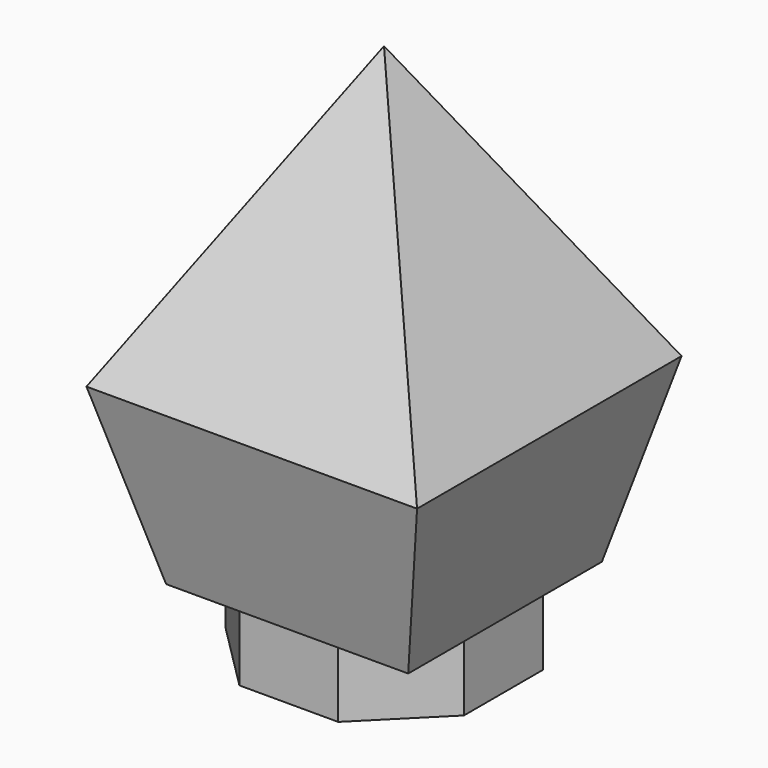
from build123d import *

# Parameters (mm, degrees)
F0_W        = 25
F0_H        = 25
F0_R        = 7.5
F1_DEPTH    = 35
F2_DEPTH    = 15
F3_SIZE2    = 21.650625
F3_SIZE     = 12.49999
F4_R        = 7.5
F5_DEPTH    = 5
F6_T1_DEPTH = 95.1228407313
F6_T3_DEPTH = 95.1228407313


# Not quite as in the source:
# - a fillet or chamfer that OpenCascade refuses, or shapes differently, is made with other operations: its cross-section is extruded or revolved along the edge and cut away or added
# - a fillet or chamfer is up to 0.001 mm smaller than in the source, because OpenCascade refuses the exact size


with BuildPart() as f1:
    # F0 (on Top) → F1 (new body)
    with BuildSketch(Plane.XY):
        with Locations((-12.5, -12.5)):
            Rectangle(F0_W, F0_H)
        with Locations((-12.5, -12.5)):
            Circle(F0_R, mode=Mode.SUBTRACT)
        with Locations((-12.5, -12.5)):
            Circle(F0_R)
    extrude(amount=F1_DEPTH)

    # F0 (on Top) → F2 (cut)
    with BuildSketch(Plane.XY):
        with Locations((-12.5, -12.5)):
            Circle(F0_R)
    extrude(amount=F2_DEPTH, mode=Mode.SUBTRACT)

    # F3 (size 12.5 and 21.6506350946 in the source; OpenCascade refuses exactly that, so slightly less here)
    f3_edges = [f1.edges().sort_by_distance(p)[0] for p in [
        (-25, -12.5, 35),
        (-12.5, -25, 35),
        (0, -12.5, 35),
        (-12.5, 0, 35),
    ]]
    f3_side = f1.faces().sort_by_distance((-12.5, -12.5, 35))[0]
    chamfer(f3_edges, length=F3_SIZE, length2=F3_SIZE2, reference=f3_side)

    # F4 (on Top) → F5 (join)
    with BuildSketch(Plane.XY):
        Polygon((-3.4594764784, -16.2579490188), (-3.4594764784, -8.802104896), (-8.731554417, -3.5300269574), (-16.1873985398, -3.5300269574), (-21.4594764784, -8.802104896), (-21.4594764784, -16.2579490188), (-16.1873985398, -21.5300269574), (-8.731554417, -21.5300269574), align=None)
        with Locations((-12.4594764784, -12.5300269574)):
            Circle(F4_R, mode=Mode.SUBTRACT)
    extrude(amount=-F5_DEPTH)

    # F6: chamfer of 13.5 x 3.3659280384 on 4 edges, made by hand

    # F6_s2 → F6_t1 (cut)
    with BuildSketch(Plane.YZ.offset(-60.0614203657)):
        Polygon((-25, 13.5), (-21.6340719616, 0), (-25, 0), align=None)
        Polygon((-3.3659280384, 0), (0, 13.5), (0, 0), align=None)
    extrude(amount=F6_T1_DEPTH, mode=Mode.SUBTRACT)

    # F6_s4 → F6_t3 (cut)
    with BuildSketch(Plane.XZ.offset(-35.0614203657)):
        Polygon((0, 13.5), (-3.3659280384, 0), (0, 0), align=None)
        Polygon((-21.6340719616, 0), (-25, 13.5), (-25, 0), align=None)
    extrude(amount=F6_T3_DEPTH, mode=Mode.SUBTRACT)


solid = f1.part
